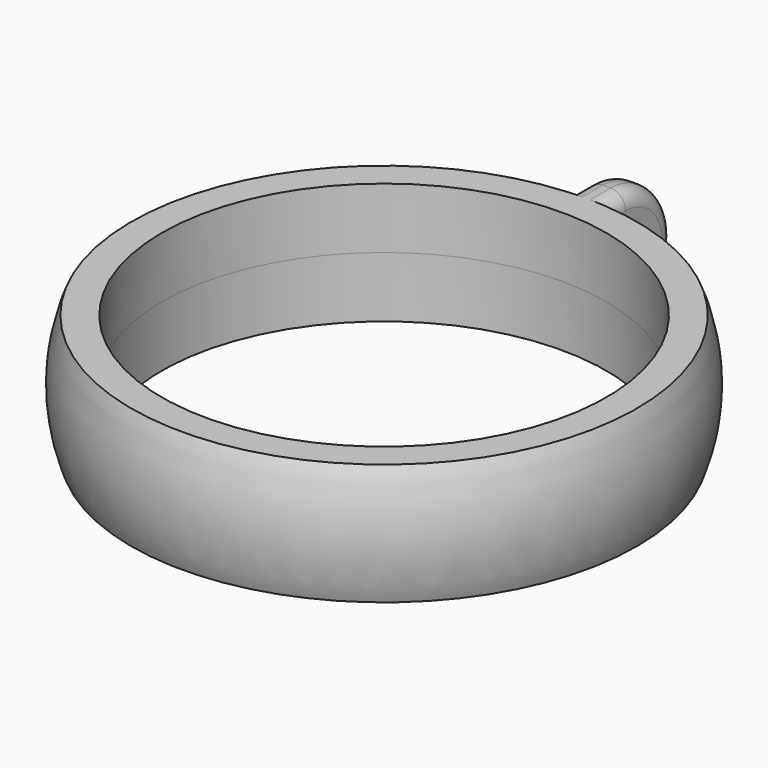
from build123d import *

# Parameters (mm, degrees)
F3_DEPTH  = 3
F4_DEPTH  = 3
F5_R      = 2.99999
F6_R      = 0.75
F8_DEPTH  = 2
F9_R      = 11
F10_DEPTH = 25


# Not quite as in the source:
# - a fillet or chamfer is up to 0.001 mm smaller than in the source, because OpenCascade refuses the exact size


with BuildPart() as f1:
    # F0 (on Front) → F1 (revolve)
    with BuildSketch(Plane.XZ):
        with BuildLine():
            Line((-11, 0), (-11, 3))
            Line((-11, 3), (-12.5, 3))
            ThreePointArc((-12.5, 3), (-13.0556042785, 0), (-12.5, -3))
            Line((-12.5, -3), (-11, -3))
            Line((-11, -3), (-11, 0))
        make_face()
    revolve(axis=Axis((0, 0, 1.9247694872), (0, 0, 1)))

    # F2 (on Top) → F3 (join)
    with BuildSketch(Plane.XY):
        with BuildLine():
            Line((0.9405623698, 12.4645634672), (0.9405623698, 16.7590089038))
            Line((0.9405623698, 16.7590089038), (-0.9405623698, 16.7590089038))
            Line((-0.9405623698, 16.7590089038), (-0.9405623698, 12.4645634672))
            ThreePointArc((-0.9405623698, 12.4645634672), (0, 12.5), (0.9405623698, 12.4645634672))
        make_face()
    extrude(amount=F3_DEPTH)

    # F3_face (on face) + F2 (on Top) → F4 (join)
    with BuildSketch(Plane(origin=(0, 14.9016416929, 0), x_dir=(1, 0, 0), z_dir=(0, 0, -1))):
        with BuildLine():
            add(Edge.make_bspline(
                [(-0.9405623698, 1.8799618663), (-0.4710967186, 1.8460521303), (0, 1.8347096394), (0.4710967186, 1.8460521303), (0.9405623698, 1.8799618663)],
                knots=[0, 0, 0, 0, 0, 1, 1, 1, 1, 1], degree=4))
            Line((-0.9405623698, 1.8799618663), (-0.9405623698, -1.8573672109))
            Line((-0.9405623698, -1.8573672109), (0.9405623698, -1.8573672109))
            Line((0.9405623698, -1.8573672109), (0.9405623698, 1.8799618663))
        make_face()
    with BuildSketch(Plane.XY):
        with BuildLine():
            Line((0.9405623698, 12.4645634672), (0.9405623698, 16.7590089038))
            Line((0.9405623698, 16.7590089038), (-0.9405623698, 16.7590089038))
            Line((-0.9405623698, 16.7590089038), (-0.9405623698, 12.4645634672))
            ThreePointArc((-0.9405623698, 12.4645634672), (0, 12.5), (0.9405623698, 12.4645634672))
        make_face()
        with BuildLine():
            ThreePointArc((12.5, 0), (9.1653431366, 8.4997932439), (0.9405623698, 12.4645634672))
            ThreePointArc((0.9405623698, 12.4645634672), (0, 12.5), (-0.9405623698, 12.4645634672))
            ThreePointArc((-0.9405623698, 12.4645634672), (-8.4997932439, -9.1653431366), (12.5, 0))
        make_face()
    extrude(amount=F4_DEPTH, dir=(0, 0, -1))

    # F5 (radius 3 in the source; OpenCascade refuses exactly that, so slightly less here)
    f5_edges = [f1.edges().sort_by_distance(p)[0] for p in [
        (0, 16.759009, 3),
        (0, 16.759009, -3),
    ]]
    fillet(f5_edges, radius=F5_R)

    # F6
    f6_edges = [f1.edges().sort_by_distance(p)[0] for p in [
        (0.940562, 13.111791, -3),
        (0.940562, 15.880332, 2.121323),
        (-0.940562, 15.880332, 2.121323),
        (-0.940562, 13.111791, 3),
        (-0.940562, 13.111791, -3),
    ]]
    fillet(f6_edges, radius=F6_R)

    # F7 (on face) → F8 (cut)
    with BuildSketch(Plane(origin=(-0.9405623698, 0, 0), x_dir=(0, -1, 0), z_dir=(-1, 0, 0))):
        with BuildLine():
            add(Edge.make_bspline(
                [(-13.0142525221, 0.3522206963), (-13.0179655917, 0.2642177815), (-13.0229178327, 0.0881074317), (-13.0229178526, -0.0881075807), (-13.01796564, -0.2642179295), (-13.0142525781, -0.352220887)],
                knots=[0.8851801326, 0.8851801326, 0.8851801326, 0.8851801326, 0.8851801326, 1, 1.1148199242, 1.1148199242, 1.1148199242, 1.1148199242, 1.1148199242], degree=4))
            ThreePointArc((-13.0142525221, 0.3522206963), (-15.4636025882, 9.94e-08), (-13.0142525781, -0.352220887))
        make_face()
    extrude(amount=-F8_DEPTH, mode=Mode.SUBTRACT)

    # F9 (on face) → F10 (cut)
    with BuildSketch(Plane.XY):
        Circle(F9_R)
    extrude(amount=-F10_DEPTH, mode=Mode.SUBTRACT)


solid = f1.part
